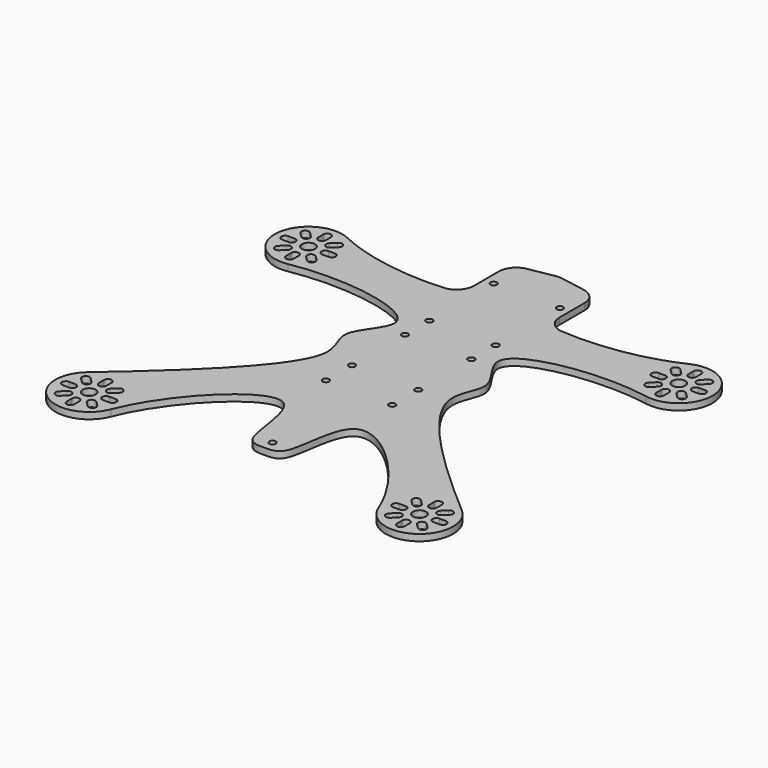
from build123d import *

# Parameters (mm, degrees)
F0_R     = 1.5
F1_DEPTH = 3
F2_R     = 8
F3_R     = 3
F4_DEPTH = 25


# Not quite as in the source:
# - a pattern or mirror of a feature is missing from the dataset's text; its kind, count and spacing are read off the source's solid
# - a feature names something its author has since deleted; it is built from what else it names


with BuildPart() as f1:
    # F0 (on Top) → F1 (new body)
    with BuildSketch(Plane.XY):
        with BuildLine():
            add(Edge.make_bspline(
                [(61.5576017777, -83.1273558257), (52.4812214136, -59.8331651447), (9.2489784273, -17.6971482628), (11.207338145, -71.121793424), (3.7947684949, -72), (0, -72)],
                knots=[0, 0, 0, 0, 0.4834491607, 0.8163929405, 1, 1, 1, 1], degree=3))
            ThreePointArc((61.5576017777, -83.1273558257), (84.929063486, -90.1697208045), (86.1564430337, -65.7911714974))
            add(Edge.make_bspline(
                [(82.4179560822, 44.9444015549), (57.8231720776, 49.4273246821), (8.3131086492, 40.384824142), (38.8189243822, 15.5137154471), (15.690189555, -4.5419342112), (67.2712357714, -49.4098117656), (86.1564430337, -65.7911714974)],
                knots=[0, 0, 0, 0, 0.2999546301, 0.4726870144, 0.6398086984, 1, 1, 1, 1], degree=3))
            ThreePointArc((82.4179560822, 44.9444015549), (100.568115037, 62.1907032369), (78.6127369102, 74.2250109902))
            add(Edge.make_bspline(
                [(19.6961550602, 66.5270364467), (29.6007581055, 64.4037500024), (55.9807315031, 63.6046375857), (78.6127369102, 74.2250109902)],
                knots=[0, 0, 0, 0, 59.4173579769, 59.4173579769, 59.4173579769, 59.4173579769], degree=3))
            Line((19.6961550602, 66.5270364467), (19.6961550602, 94.5270364467))
            Line((19.6961550602, 94.5270364467), (0, 98))
            Line((0, 98), (-19.6961550602, 94.5270364467))
            Line((-19.6961550602, 94.5270364467), (-19.6961550602, 66.5270364467))
            add(Edge.make_bspline(
                [(-19.6961550602, 66.5270364467), (-29.6007581055, 64.4037500024), (-55.9807315031, 63.6046375857), (-78.6127369102, 74.2250109902)],
                knots=[0, 0, 0, 0, 59.4173579769, 59.4173579769, 59.4173579769, 59.4173579769], degree=3))
            ThreePointArc((-78.6127369102, 74.2250109902), (-100.568115037, 62.1907032369), (-82.4179560822, 44.9444015549))
            add(Edge.make_bspline(
                [(-82.4179560822, 44.9444015549), (-57.8231720776, 49.4273246821), (-8.3131086492, 40.384824142), (-38.8189243822, 15.5137154471), (-15.690189555, -4.5419342112), (-67.2712357714, -49.4098117656), (-86.1564430337, -65.7911714974)],
                knots=[0, 0, 0, 0, 0.2999546301, 0.4726870144, 0.6398086984, 1, 1, 1, 1], degree=3))
            ThreePointArc((-86.1564430337, -65.7911714974), (-84.929063486, -90.1697208045), (-61.5576017777, -83.1273558257))
            add(Edge.make_bspline(
                [(-61.5576017777, -83.1273558257), (-52.4812214136, -59.8331651447), (-9.2489784273, -17.6971482628), (-11.207338145, -71.121793424), (-3.7947684949, -72), (0, -72)],
                knots=[0, 0, 0, 0, 0.4834491607, 0.8163929405, 1, 1, 1, 1], degree=3))
        make_face()
        with Locations((0, -67)):
            Circle(F0_R, mode=Mode.SUBTRACT)
        with Locations((-15.25, -17.25)):
            Circle(F0_R, mode=Mode.SUBTRACT)
        with Locations((-15.25, -2.25)):
            Circle(F0_R, mode=Mode.SUBTRACT)
        with Locations((15.25, -17.25)):
            Circle(F0_R, mode=Mode.SUBTRACT)
        with Locations((15.25, -2.25)):
            Circle(F0_R, mode=Mode.SUBTRACT)
        with Locations((-15.25, 28.25)):
            Circle(F0_R, mode=Mode.SUBTRACT)
        with Locations((-15.25, 42.25)):
            Circle(F0_R, mode=Mode.SUBTRACT)
        with Locations((-15.25, 79.25)):
            Circle(F0_R, mode=Mode.SUBTRACT)
        with Locations((15.25, 28.25)):
            Circle(F0_R, mode=Mode.SUBTRACT)
        with Locations((15.25, 42.25)):
            Circle(F0_R, mode=Mode.SUBTRACT)
        with Locations((15.25, 79.25)):
            Circle(F0_R, mode=Mode.SUBTRACT)
    extrude(amount=F1_DEPTH)

    # F2
    f2_edges = [f1.edges().sort_by_distance(p)[0] for p in [
        (-19.696155, 66.527036, 1.5),
        (-19.696155, 94.527036, 1.5),
        (19.696155, 66.527036, 1.5),
        (19.696155, 94.527036, 1.5),
        (0, 98, 1.5),
    ]]
    fillet(f2_edges, radius=F2_R)

    # F3 (on face) → F4 (cut)
    with BuildSketch(Plane.XY.offset(3)):
        with Locations((-85.1973684211, 60.1931676378)):
            Circle(F3_R)
        with BuildLine():
            ThreePointArc((-83.4473684211, 70.9431676378), (-85.1973684211, 72.6931676378), (-86.9473684211, 70.9431676378))
            Line((-86.9473684211, 70.9431676378), (-86.9473684211, 67.9431676378))
            ThreePointArc((-86.9473684211, 67.9431676378), (-85.1973684211, 66.1931676378), (-83.4473684211, 67.9431676378))
            Line((-83.4473684211, 67.9431676378), (-83.4473684211, 70.9431676378))
        make_face()
        with BuildLine():
            ThreePointArc((-91.5613294517, 69.0320024026), (-94.0362031859, 69.0320024026), (-94.0362031859, 66.5571286685))
            Line((-94.0362031859, 66.5571286685), (-91.9148828423, 64.4358083249))
            ThreePointArc((-91.9148828423, 64.4358083249), (-89.4400091082, 64.4358083249), (-89.4400091082, 66.9106820591))
            Line((-89.4400091082, 66.9106820591), (-91.5613294517, 69.0320024026))
        make_face()
        with BuildLine():
            ThreePointArc((-95.9473684211, 61.9431676378), (-97.6973684211, 60.1931676378), (-95.9473684211, 58.4431676378))
            Line((-95.9473684211, 58.4431676378), (-92.9473684211, 58.4431676378))
            ThreePointArc((-92.9473684211, 58.4431676378), (-91.1973684211, 60.1931676378), (-92.9473684211, 61.9431676378))
            Line((-92.9473684211, 61.9431676378), (-95.9473684211, 61.9431676378))
        make_face()
        with BuildLine():
            ThreePointArc((-94.0362031859, 53.8292066071), (-94.0362031859, 51.354332873), (-91.5613294517, 51.354332873))
            Line((-91.5613294517, 51.354332873), (-89.4400091082, 53.4756532165))
            ThreePointArc((-89.4400091082, 53.4756532165), (-89.4400091082, 55.9505269507), (-91.9148828423, 55.9505269507))
            Line((-91.9148828423, 55.9505269507), (-94.0362031859, 53.8292066071))
        make_face()
        with BuildLine():
            ThreePointArc((-86.9473684211, 49.4431676378), (-85.1973684211, 47.6931676378), (-83.4473684211, 49.4431676378))
            Line((-83.4473684211, 49.4431676378), (-83.4473684211, 52.4431676378))
            ThreePointArc((-83.4473684211, 52.4431676378), (-85.1973684211, 54.1931676378), (-86.9473684211, 52.4431676378))
            Line((-86.9473684211, 52.4431676378), (-86.9473684211, 49.4431676378))
        make_face()
        with BuildLine():
            ThreePointArc((-78.8334073904, 51.354332873), (-76.3585336562, 51.354332873), (-76.3585336562, 53.8292066071))
            Line((-76.3585336562, 53.8292066071), (-78.4798539998, 55.9505269507))
            ThreePointArc((-78.4798539998, 55.9505269507), (-80.9547277339, 55.9505269507), (-80.9547277339, 53.4756532165))
            Line((-80.9547277339, 53.4756532165), (-78.8334073904, 51.354332873))
        make_face()
        with BuildLine():
            ThreePointArc((-74.4473684211, 58.4431676378), (-72.6973684211, 60.1931676378), (-74.4473684211, 61.9431676378))
            Line((-74.4473684211, 61.9431676378), (-77.4473684211, 61.9431676378))
            ThreePointArc((-77.4473684211, 61.9431676378), (-79.1973684211, 60.1931676378), (-77.4473684211, 58.4431676378))
            Line((-77.4473684211, 58.4431676378), (-74.4473684211, 58.4431676378))
        make_face()
        with BuildLine():
            ThreePointArc((-76.3585336562, 66.5571286685), (-76.3585336562, 69.0320024026), (-78.8334073904, 69.0320024026))
            Line((-78.8334073904, 69.0320024026), (-80.9547277339, 66.9106820591))
            ThreePointArc((-80.9547277339, 66.9106820591), (-80.9547277339, 64.4358083249), (-78.4798539998, 64.4358083249))
            Line((-78.4798539998, 64.4358083249), (-76.3585336562, 66.5571286685))
        make_face()
        with Locations((-76, -77.5)):
            Circle(F3_R)
        with BuildLine():
            ThreePointArc((-74.25, -66.75), (-76, -65), (-77.75, -66.75))
            Line((-77.75, -66.75), (-77.75, -69.75))
            ThreePointArc((-77.75, -69.75), (-76, -71.5), (-74.25, -69.75))
            Line((-74.25, -69.75), (-74.25, -66.75))
        make_face()
        with BuildLine():
            ThreePointArc((-82.3639610307, -68.6611652352), (-84.8388347648, -68.6611652352), (-84.8388347648, -71.1360389693))
            Line((-84.8388347648, -71.1360389693), (-82.7175144213, -73.2573593129))
            ThreePointArc((-82.7175144213, -73.2573593129), (-80.2426406871, -73.2573593129), (-80.2426406871, -70.7824855787))
            Line((-80.2426406871, -70.7824855787), (-82.3639610307, -68.6611652352))
        make_face()
        with BuildLine():
            ThreePointArc((-86.75, -75.75), (-88.5, -77.5), (-86.75, -79.25))
            Line((-86.75, -79.25), (-83.75, -79.25))
            ThreePointArc((-83.75, -79.25), (-82, -77.5), (-83.75, -75.75))
            Line((-83.75, -75.75), (-86.75, -75.75))
        make_face()
        with BuildLine():
            ThreePointArc((-84.8388347648, -83.8639610307), (-84.8388347648, -86.3388347648), (-82.3639610307, -86.3388347648))
            Line((-82.3639610307, -86.3388347648), (-80.2426406871, -84.2175144213))
            ThreePointArc((-80.2426406871, -84.2175144213), (-80.2426406871, -81.7426406871), (-82.7175144213, -81.7426406871))
            Line((-82.7175144213, -81.7426406871), (-84.8388347648, -83.8639610307))
        make_face()
        with BuildLine():
            ThreePointArc((-77.75, -88.25), (-76, -90), (-74.25, -88.25))
            Line((-74.25, -88.25), (-74.25, -85.25))
            ThreePointArc((-74.25, -85.25), (-76, -83.5), (-77.75, -85.25))
            Line((-77.75, -85.25), (-77.75, -88.25))
        make_face()
        with BuildLine():
            ThreePointArc((-69.6360389693, -86.3388347648), (-67.1611652352, -86.3388347648), (-67.1611652352, -83.8639610307))
            Line((-67.1611652352, -83.8639610307), (-69.2824855787, -81.7426406871))
            ThreePointArc((-69.2824855787, -81.7426406871), (-71.7573593129, -81.7426406871), (-71.7573593129, -84.2175144213))
            Line((-71.7573593129, -84.2175144213), (-69.6360389693, -86.3388347648))
        make_face()
        with BuildLine():
            ThreePointArc((-65.25, -79.25), (-63.5, -77.5), (-65.25, -75.75))
            Line((-65.25, -75.75), (-68.25, -75.75))
            ThreePointArc((-68.25, -75.75), (-70, -77.5), (-68.25, -79.25))
            Line((-68.25, -79.25), (-65.25, -79.25))
        make_face()
        with BuildLine():
            ThreePointArc((-67.1611652352, -71.1360389693), (-67.1611652352, -68.6611652352), (-69.6360389693, -68.6611652352))
            Line((-69.6360389693, -68.6611652352), (-71.7573593129, -70.7824855787))
            ThreePointArc((-71.7573593129, -70.7824855787), (-71.7573593129, -73.2573593129), (-69.2824855787, -73.2573593129))
            Line((-69.2824855787, -73.2573593129), (-67.1611652352, -71.1360389693))
        make_face()
    f4 = extrude(amount=-F4_DEPTH, mode=Mode.SUBTRACT)

    # F4_copies: F4 across plane
    add(f4.mirror(Plane(origin=(0, 0, 0), x_dir=(0, 0, 1), z_dir=(1, 0, 0))), mode=Mode.SUBTRACT)


solid = f1.part
